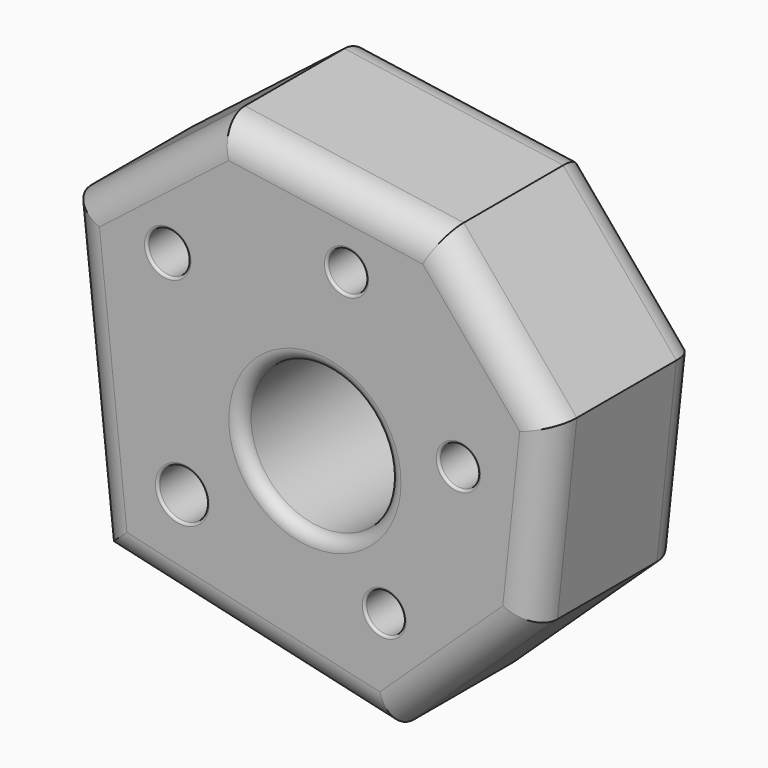
from build123d import *

# Parameters (mm, degrees)
F0_R         = 4.994353159
F0_R_2       = 3.9756540209
F0_R_3       = 15.0575134539
F0_R_4       = 4.2314308146
F0_R_5       = 4.0142888821
F0_R_6       = 4.0065925918
F1_DEPTH     = 38.1
F2_T1_DEPTH  = 76.9402628143
F2_T3_DEPTH  = 67.7321934705
F2_T5_DEPTH  = 69.4802582589
F2_T7_DEPTH  = 72.0042494327
F2_T9_DEPTH  = 92.6885025387
F2_T11_DEPTH = 93.2161117618
F2_T13_DEPTH = 71.4132355611
F3_R         = 2.54
F4_R         = 0.508


# Not quite as in the source:
# - a fillet or chamfer that OpenCascade refuses, or shapes differently, is made with other operations: its cross-section is extruded or revolved along the edge and cut away or added


with BuildPart() as f1:
    # F0 (on Front) → F1 (new body)
    with BuildSketch(Plane.XZ):
        Polygon((-50.6895668805, 28.8208909333), (-44.229131192, -32.3047637939), (15.157174319, -45.9710657597), (44.4776155055, -18.3899793774), (48.4532564878, 19.1302374005), (25.3447815776, 46.7113293707), (-19.3813033402, 53.1717613339), align=None)
        with Locations((-27.0841307938, -16.6506320238)):
            Circle(F0_R, mode=Mode.SUBTRACT)
        with Locations((14.1632612795, -24.6019363403)):
            Circle(F0_R_2, mode=Mode.SUBTRACT)
        Circle(F0_R_3, mode=Mode.SUBTRACT)
        with Locations((-30.0658699125, 25.8391518146)):
            Circle(F0_R_4, mode=Mode.SUBTRACT)
        with Locations((29.3204355985, 6.706325803)):
            Circle(F0_R_5, mode=Mode.SUBTRACT)
        with Locations((6.4604342915, 34.2874154449)):
            Circle(F0_R_6, mode=Mode.SUBTRACT)
    extrude(amount=-F1_DEPTH)

    # F2: fillet of radius 6.35 on 20 edges, made by hand

    # F2_s2 → F2_t1 (cut)
    with BuildSketch(Plane(origin=(33.9294367843, 0, -4.9009167312), x_dir=(0, 1, 0), z_dir=(-0.9897283647, 0, 0.1429607079))):
        with BuildLine():
            ThreePointArc((6.35, -49.8548355499), (1.8598719395, -47.9949636104), (0, -43.5048355499))
            Line((0, -43.5048355499), (0, -49.8548355499))
            Line((0, -49.8548355499), (6.35, -49.8548355499))
        make_face()
        with BuildLine():
            ThreePointArc((31.75, -49.8548355499), (36.2401280605, -47.9949636104), (38.1, -43.5048355499))
            Line((38.1, -43.5048355499), (38.1, -49.8548355499))
            Line((38.1, -49.8548355499), (31.75, -49.8548355499))
        make_face()
    extrude(amount=F2_T1_DEPTH, mode=Mode.SUBTRACT)

    # F2_s4 → F2_t3 (cut)
    with BuildSketch(Plane(origin=(20.7622686455, 0, -24.780780352), x_dir=(0, 1, 0), z_dir=(-0.6422197393, 0, 0.7665205845))):
        with BuildLine():
            ThreePointArc((6.35, -49.4262345597), (1.8598719395, -47.5663626202), (0, -43.0762345597))
            Line((0, -43.0762345597), (0, -49.4262345597))
            Line((0, -49.4262345597), (6.35, -49.4262345597))
        make_face()
        with BuildLine():
            ThreePointArc((31.75, -49.4262345597), (36.2401280605, -47.5663626202), (38.1, -43.0762345597))
            Line((38.1, -43.0762345597), (38.1, -49.4262345597))
            Line((38.1, -49.4262345597), (31.75, -49.4262345597))
        make_face()
    extrude(amount=F2_T3_DEPTH, mode=Mode.SUBTRACT)

    # F2_s6 → F2_t5 (cut)
    with BuildSketch(Plane(origin=(-3.1058882585, 0, -29.3119024738), x_dir=(0, 1, 0), z_dir=(0.1053700973, 0, 0.994433076))):
        with BuildLine():
            ThreePointArc((6.35, -46.167765915), (1.8598719395, -44.3078939755), (0, -39.817765915))
            Line((0, -39.817765915), (0, -46.167765915))
            Line((0, -46.167765915), (6.35, -46.167765915))
        make_face()
        with BuildLine():
            ThreePointArc((31.75, -46.167765915), (36.2401280605, -44.3078939755), (38.1, -39.817765915))
            Line((38.1, -39.817765915), (38.1, -46.167765915))
            Line((38.1, -46.167765915), (31.75, -46.167765915))
        make_face()
    extrude(amount=F2_T5_DEPTH, mode=Mode.SUBTRACT)

    # F2_s8 → F2_t7 (cut)
    with BuildSketch(Plane(origin=(-26.4641944584, 0, -24.8942786623), x_dir=(0, 1, 0), z_dir=(0.7283812666, 0, 0.6851720445))):
        with BuildLine():
            ThreePointArc((6.35, -43.8697352198), (1.8598719395, -42.0098632804), (0, -37.5197352198))
            Line((0, -37.5197352198), (0, -43.8697352198))
            Line((0, -43.8697352198), (6.35, -43.8697352198))
        make_face()
        with BuildLine():
            ThreePointArc((31.75, -43.8697352198), (36.2401280605, -42.0098632804), (38.1, -37.5197352198))
            Line((38.1, -37.5197352198), (38.1, -43.8697352198))
            Line((38.1, -43.8697352198), (31.75, -43.8697352198))
        make_face()
    extrude(amount=F2_T7_DEPTH, mode=Mode.SUBTRACT)

    # F2_s10 → F2_t9 (cut)
    with BuildSketch(Plane(origin=(-50.4150448083, 0, 11.6017863047), x_dir=(0, 1, 0), z_dir=(0.9745284678, 0, -0.2242638299))):
        with BuildLine():
            ThreePointArc((6.35, -41.4009063166), (1.8598719395, -39.5410343771), (0, -35.0509063166))
            Line((0, -35.0509063166), (0, -41.4009063166))
            Line((0, -41.4009063166), (6.35, -41.4009063166))
        make_face()
        with BuildLine():
            ThreePointArc((31.75, -41.4009063166), (36.2401280605, -39.5410343771), (38.1, -35.0509063166))
            Line((38.1, -35.0509063166), (38.1, -41.4009063166))
            Line((38.1, -41.4009063166), (31.75, -41.4009063166))
        make_face()
    extrude(amount=F2_T9_DEPTH, mode=Mode.SUBTRACT)

    # F2_s12 → F2_t11 (cut)
    with BuildSketch(Plane(origin=(-5.2409896197, 0, 49.5878199815), x_dir=(0, 1, 0), z_dir=(0.105105651, 0, -0.9944610611))):
        with BuildLine():
            ThreePointArc((6.35, -47.3795619663), (1.8598719395, -45.5196900269), (0, -41.0295619663))
            Line((0, -41.0295619663), (0, -47.3795619663))
            Line((0, -47.3795619663), (6.35, -47.3795619663))
        make_face()
        with BuildLine():
            ThreePointArc((31.75, -47.3795619663), (36.2401280605, -45.5196900269), (38.1, -41.0295619663))
            Line((38.1, -41.0295619663), (38.1, -47.3795619663))
            Line((38.1, -47.3795619663), (31.75, -47.3795619663))
        make_face()
    extrude(amount=F2_T11_DEPTH, mode=Mode.SUBTRACT)

    # F2_s14 → F2_t13 (cut)
    with BuildSketch(Plane(origin=(26.2227766231, 0, 20.395491889), x_dir=(0, 1, 0), z_dir=(-0.7893522325, 0, -0.613940594))):
        with BuildLine():
            ThreePointArc((6.35, -53.8702174028), (1.8598719395, -52.0103454633), (0, -47.5202174028))
            Line((0, -47.5202174028), (0, -53.8702174028))
            Line((0, -53.8702174028), (6.35, -53.8702174028))
        make_face()
        with BuildLine():
            ThreePointArc((31.75, -53.8702174028), (36.2401280605, -52.0103454633), (38.1, -47.5202174028))
            Line((38.1, -47.5202174028), (38.1, -53.8702174028))
            Line((38.1, -53.8702174028), (31.75, -53.8702174028))
        make_face()
    extrude(amount=F2_T13_DEPTH, mode=Mode.SUBTRACT)

    # F2_s15 → F2_t16 (revolve, cut)
    with BuildSketch(Plane.XY.offset(-16.6506320238)):
        with BuildLine():
            ThreePointArc((-22.0897776348, 31.75), (-20.2299056954, 36.2401280605), (-15.7397776348, 38.1))
            Line((-15.7397776348, 38.1), (-22.0897776348, 38.1))
            Line((-22.0897776348, 38.1), (-22.0897776348, 31.75))
        make_face()
    revolve(axis=Axis((-27.0841307938, 38.1, -16.6506320238), (0, -1, 0)), mode=Mode.SUBTRACT)

    # F2_s17 → F2_t18 (revolve, cut)
    with BuildSketch(Plane.XY.offset(-24.6019363403)):
        with BuildLine():
            ThreePointArc((18.1389153004, 31.75), (19.9987872398, 36.2401280605), (24.4889153004, 38.1))
            Line((24.4889153004, 38.1), (18.1389153004, 38.1))
            Line((18.1389153004, 38.1), (18.1389153004, 31.75))
        make_face()
    revolve(axis=Axis((14.1632612795, 38.1, -24.6019363403), (0, -1, 0)), mode=Mode.SUBTRACT)

    # F2_s19 → F2_t20 (revolve, cut)
    with BuildSketch(Plane.XY):
        with BuildLine():
            ThreePointArc((15.0575134539, 31.75), (16.9173853934, 36.2401280605), (21.4075134539, 38.1))
            Line((21.4075134539, 38.1), (15.0575134539, 38.1))
            Line((15.0575134539, 38.1), (15.0575134539, 31.75))
        make_face()
    revolve(axis=Axis((0, 38.1, 0), (0, -1, 0)), mode=Mode.SUBTRACT)

    # F2_s21 → F2_t22 (revolve, cut)
    with BuildSketch(Plane.XY.offset(25.8391518146)):
        with BuildLine():
            ThreePointArc((-25.8344390979, 31.75), (-23.9745671584, 36.2401280605), (-19.4844390979, 38.1))
            Line((-19.4844390979, 38.1), (-25.8344390979, 38.1))
            Line((-25.8344390979, 38.1), (-25.8344390979, 31.75))
        make_face()
    revolve(axis=Axis((-30.0658699125, 38.1, 25.8391518146), (0, -1, 0)), mode=Mode.SUBTRACT)

    # F2_s23 → F2_t24 (revolve, cut)
    with BuildSketch(Plane.XY.offset(6.706325803)):
        with BuildLine():
            ThreePointArc((33.3347244806, 31.75), (35.1945964201, 36.2401280605), (39.6847244806, 38.1))
            Line((39.6847244806, 38.1), (33.3347244806, 38.1))
            Line((33.3347244806, 38.1), (33.3347244806, 31.75))
        make_face()
    revolve(axis=Axis((29.3204355985, 38.1, 6.706325803), (0, -1, 0)), mode=Mode.SUBTRACT)

    # F2_s25 → F2_t26 (revolve, cut)
    with BuildSketch(Plane.XY.offset(34.2874154449)):
        with BuildLine():
            ThreePointArc((10.4670268833, 31.75), (12.3268988228, 36.2401280605), (16.8170268833, 38.1))
            Line((16.8170268833, 38.1), (10.4670268833, 38.1))
            Line((10.4670268833, 38.1), (10.4670268833, 31.75))
        make_face()
    revolve(axis=Axis((6.4604342915, 38.1, 34.2874154449), (0, -1, 0)), mode=Mode.SUBTRACT)

    # F3
    f3_edges = [f1.edges().sort_by_distance(p)[0] for p in [
        (-15.057513, 0, 0),
        (-15.057513, 31.75, 0),
    ]]
    fillet(f3_edges, radius=F3_R)

    # F4
    f4_edges = [f1.edges().sort_by_distance(p)[0] for p in [
        (-34.297301, 0, 25.839152),
        (2.453842, 0, 34.287415),
        (25.306147, 0, 6.706326),
        (10.187607, 0, -24.601936),
        (-32.078484, 0, -16.650632),
    ]]
    fillet(f4_edges, radius=F4_R)


solid = f1.part
